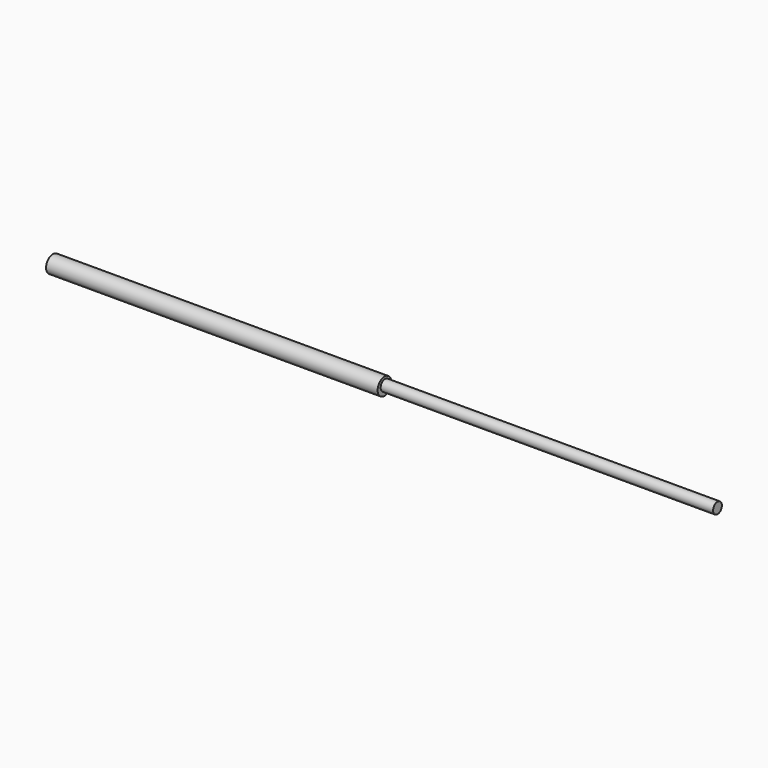
from build123d import *

# Parameters (mm, degrees)
F0_R     = 65.6478190294
F1_DEPTH = 1270
F2_R     = 42.2688566602
F3_DEPTH = 2546.7877856


# Not quite as in the source:
# - an extrude ends at something that could not be found from the text; its depth is read off the source's solid


with BuildPart() as f1:
    # F0 (on Right) → F1 (new body, symmetric)
    with BuildSketch(Plane.YZ):
        Circle(F0_R)
    extrude(amount=F1_DEPTH, both=True)

    # F2 (on face) → F3 (join, through all)
    with BuildSketch(Plane.YZ.offset(1270)):
        with Locations((5.3433440626, 5.0906497054)):
            Circle(F2_R)
    extrude(amount=F3_DEPTH)


solid = f1.part
